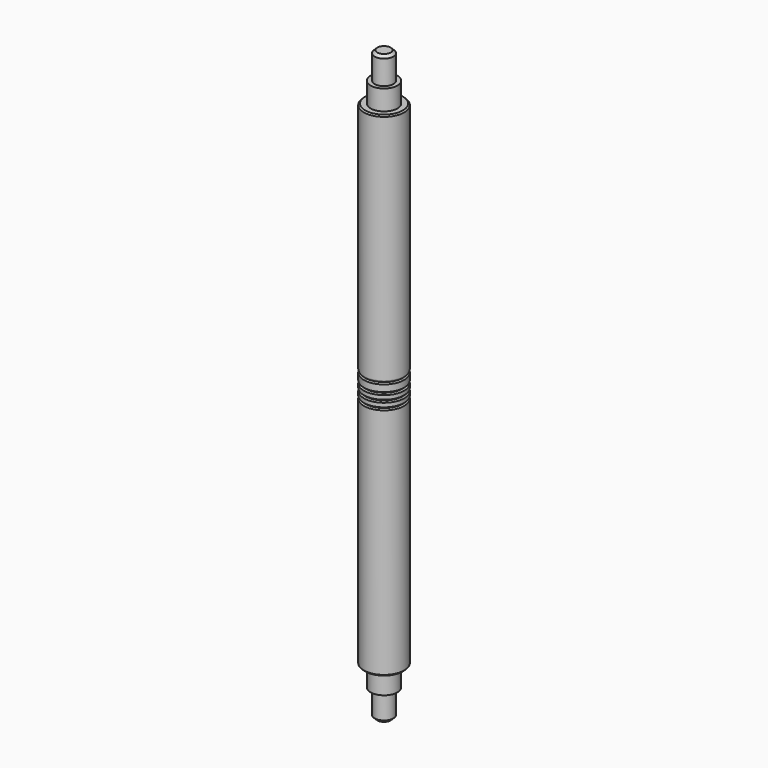
from build123d import *

# Parameters (mm, degrees)
F0_W     = 0.7
F0_H     = 2
F2_SIZE2 = 0.2
F2_SIZE  = 0.2
F3_SIZE2 = 0.1
F3_SIZE  = 0.1
F4_SIZE2 = 0.2
F4_SIZE  = 0.2


# Not quite as in the source:
# - a fillet or chamfer that OpenCascade refuses, or shapes differently, is made with other operations: its cross-section is extruded or revolved along the edge and cut away or added


with BuildPart() as f1:
    # F0 (on Front) → F1 (revolve)
    with BuildSketch(Plane.XZ):
        Polygon((0, 38.25), (0, 36.75), (1, 36.75), (1, 38.25), (0.7, 38.25), align=None)
        Polygon((1, 36.75), (0, 36.75), (0, 0), (1, 0), (1.5, 0), (1.5, 17.425), (1.4, 17.525), (1.5, 17.625), (1.5, 17.925), (1.4, 18.025), (1.5, 18.125), (1.5, 18.425), (1.4, 18.525), (1.5, 18.625), (1.5, 19.125), (1.4, 19.225), (1.5, 19.325), (1.5, 36.75), align=None)
        with Locations((0.35, 39.25)):
            Rectangle(F0_W, F0_H)
        Polygon((1, 0), (0, 0), (0, -1.5), (0.7, -1.5), (1, -1.5), align=None)
        with Locations((0.35, -2.5)):
            Rectangle(F0_W, F0_H)
    revolve(axis=Axis((0, 0, 18.375), (0, 0, -1)))

    # F2
    f2_edges = [f1.edges().sort_by_distance(p)[0] for p in [
        (-0.7, 0, 40.25),
    ]]
    chamfer(f2_edges, length=F2_SIZE, length2=F2_SIZE2)

    # F3
    f3_edges = [f1.edges().sort_by_distance(p)[0] for p in [
        (-1.5, 0, 36.75),
    ]]
    chamfer(f3_edges, length=F3_SIZE, length2=F3_SIZE2)

    # F4
    f4_edges = [f1.edges().sort_by_distance(p)[0] for p in [
        (-0.7, 0, -3.5),
    ]]
    chamfer(f4_edges, length=F4_SIZE, length2=F4_SIZE2)

    # F5: chamfer of 0.1 on 2 edges, made by hand

    # F5_s1 → F5_t2 (revolve, cut)
    with BuildSketch(Plane.XZ):
        Polygon((1.4, 0), (1.5, 0.1), (1.5, 0), align=None)
    revolve(axis=Axis((0, 0, 0), (0, 0, -1)), mode=Mode.SUBTRACT)

    # F5_s3 → F5_t4 (revolve, cut)
    with BuildSketch(Plane.XZ):
        Polygon((1.4707106781, 19.2957106781), (1.5, 19.3664213562), (1.5, 19.325), align=None)
    revolve(axis=Axis((0, 0, 19.325), (0, 0, -1)), mode=Mode.SUBTRACT)


solid = f1.part
